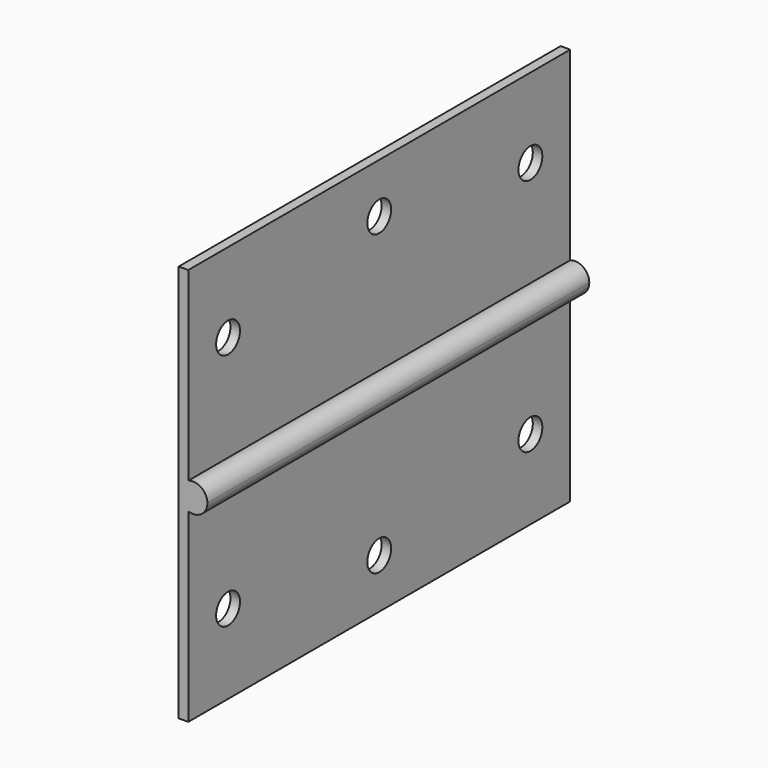
from build123d import *

# Parameters (mm, degrees)
F0_W     = 76.2
F0_H     = 63.5
F1_DEPTH = 1.524
F3_DEPTH = 76.2
F5_D     = 4.7625


# Not quite as in the source:
# - a pattern or mirror of a feature is missing from the dataset's text; its kind, count and spacing are read off the source's solid


with BuildPart() as f1:
    # F0 (on Right) → F1 (new body)
    with BuildSketch(Plane.YZ):
        Rectangle(F0_W, F0_H)
    extrude(amount=F1_DEPTH)

    # F2 (on face) → F3 (join, through all)
    with BuildSketch(Plane.XZ.offset(38.1)):
        with BuildLine():
            ThreePointArc((1.524, -2.1552614691), (3.6058227154, -1.866511184), (4.572, 0))
            ThreePointArc((4.572, 0), (3.6058227154, 1.866511184), (1.524, 2.1552614691))
            Line((1.524, 2.1552614691), (1.524, -2.1552614691))
        make_face()
    extrude(amount=-F3_DEPTH)

    # F5 (through all)
    with Locations(Plane.YZ.offset(1.524)):
        with Locations((-30.1625, 19.05), (0, 23.8125), (30.1625, 19.05)):
            f5 = Hole(F5_D / 2)

    # F5_copies: F5 across plane
    add(f5.mirror(Plane(origin=(0, 0, 0), x_dir=(-1, 0, 0), z_dir=(0, 0, -1))), mode=Mode.SUBTRACT)


solid = f1.part
